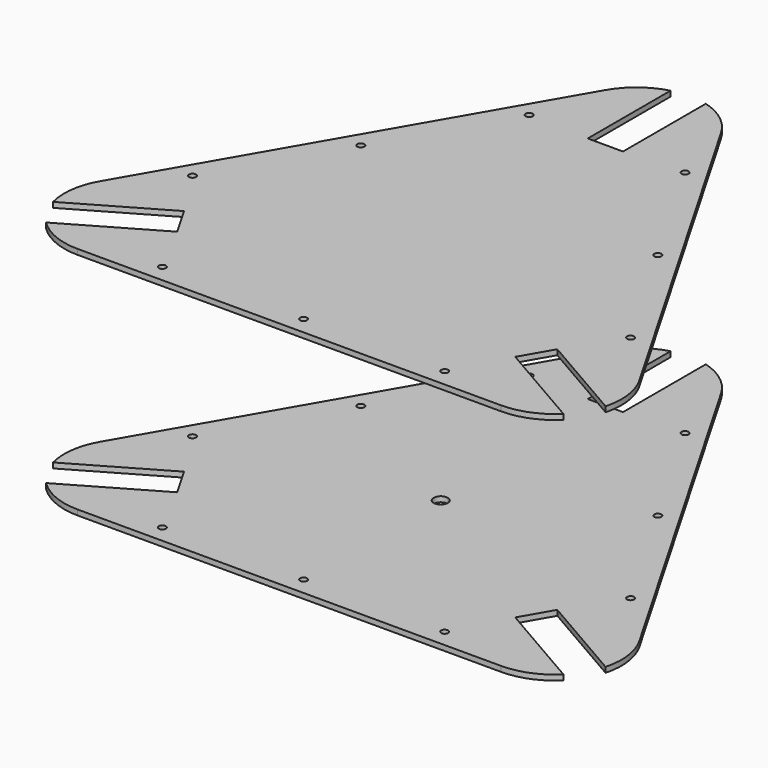
from build123d import *

# Parameters (mm, degrees)
F0_R     = 2
F0_R_2   = 4
F0_W     = 240
F0_H     = 20
F1_DEPTH = 3
F3_DEPTH = 3


# Not quite as in the source:
# - a feature names something its author has since deleted; it is built from what else it names


with BuildPart() as f1:
    # F0 (on Top) → F1 (new body)
    with BuildSketch(Plane.XY):
        Polygon((135.5000008485, -60.3331046), (152.8205089242, -50.3331046), (32.8205089242, 157.5129923082), (15.5000008485, 147.5129923082), align=None)
        with Locations((124.1602548864, -20.6920884487)):
            Circle(F0_R, mode=Mode.SUBTRACT)
        with Locations((84.1602548864, 48.5899438541)):
            Circle(F0_R, mode=Mode.SUBTRACT)
        with Locations((44.1602548864, 117.8719761568)):
            Circle(F0_R, mode=Mode.SUBTRACT)
        Polygon((-32.8205072271, 157.5129952477), (-152.8205072271, -50.3331016606), (-135.4999991515, -60.3331016606), (-15.4999991515, 147.5129952477), align=None)
        with Locations((-124.1602531893, -20.6920855092)):
            Circle(F0_R, mode=Mode.SUBTRACT)
        with Locations((-84.1602531893, 48.5899467935)):
            Circle(F0_R, mode=Mode.SUBTRACT)
        with Locations((-44.1602531893, 117.8719790963)):
            Circle(F0_R, mode=Mode.SUBTRACT)
        with BuildLine():
            Line((-120.0000016971, -107.1798906476), (-120.0000016971, -87.1798906476))
            Line((-120.0000016971, -87.1798906476), (119.9999983029, -87.1798906476))
            Line((119.9999983029, -87.1798906476), (119.9999983029, -107.1798906476))
            ThreePointArc((119.9999983029, -107.1798906476), (134.3544122401, -104.3562188159), (146.5698048192, -96.3059699854))
            Line((146.5698048192, -96.3059699854), (95.7997276302, -66.9938522536))
            Line((95.7997276302, -66.9938522536), (105.7997276302, -49.6733441779))
            Line((105.7997276302, -49.6733441779), (156.6259599909, -79.0178831132))
            ThreePointArc((156.6259599909, -79.0178831132), (157.5686990784, -64.2980017881), (152.8205089242, -50.3331046))
            Line((152.8205089242, -50.3331046), (135.5000008485, -60.3331046))
            Line((135.5000008485, -60.3331046), (15.5000008485, 147.5129923082))
            Line((15.5000008485, 147.5129923082), (32.8205089242, 157.5129923082))
            ThreePointArc((32.8205089242, 157.5129923082), (23.1979304174, 168.5324435184), (10.1185141338, 175.0861593938))
            Line((10.1185141338, 175.0861593938), (10.1185141338, 116.4619239302))
            Line((10.1185141338, 116.4619239302), (-9.8814858662, 116.4619239302))
            Line((-9.8814858662, 116.4619239302), (-9.8814858662, 175.1510018008))
            ThreePointArc((-9.8814858662, 175.1510018008), (-23.1006465781, 168.6074971372), (-32.8205072271, 157.5129952477))
            Line((-32.8205072271, 157.5129952477), (-15.4999991515, 147.5129952477))
            Line((-15.4999991515, 147.5129952477), (-135.4999991515, -60.3331016606))
            Line((-135.4999991515, -60.3331016606), (-152.8205072271, -50.3331016606))
            ThreePointArc((-152.8205072271, -50.3331016606), (-157.5523414703, -64.1762244295), (-156.6883173198, -78.7801884655))
            Line((-156.6883173198, -78.7801884655), (-105.9182417641, -49.4680716766))
            Line((-105.9182417641, -49.4680716766), (-95.9182417641, -66.7885797523))
            Line((-95.9182417641, -66.7885797523), (-146.7444724884, -96.1331177429))
            ThreePointArc((-146.7444724884, -96.1331177429), (-134.4680516673, -104.3094944517), (-120.0000016971, -107.1798906476))
        make_face()
        Circle(F0_R_2, mode=Mode.SUBTRACT)
        with Locations((-1.6971e-06, -97.1798906476)):
            Rectangle(F0_W, F0_H)
        with Locations((-80.0000016971, -97.1798906476)):
            Circle(F0_R, mode=Mode.SUBTRACT)
        with Locations((-1.6971e-06, -97.1798906476)):
            Circle(F0_R, mode=Mode.SUBTRACT)
        with Locations((79.9999983029, -97.1798906476)):
            Circle(F0_R, mode=Mode.SUBTRACT)
    extrude(amount=F1_DEPTH)


with BuildPart() as f1_1:
    # F2: moved
    add(f1.part.moved(Location((0, 0, -130))))


with BuildPart() as f3:
    # F0 (on Top) → F3 (new body)
    with BuildSketch(Plane.XY):
        with BuildLine():
            Line((-120.0000016971, -107.1798906476), (-120.0000016971, -87.1798906476))
            Line((-120.0000016971, -87.1798906476), (119.9999983029, -87.1798906476))
            Line((119.9999983029, -87.1798906476), (119.9999983029, -107.1798906476))
            ThreePointArc((119.9999983029, -107.1798906476), (134.3544122401, -104.3562188159), (146.5698048192, -96.3059699854))
            Line((146.5698048192, -96.3059699854), (95.7997276302, -66.9938522536))
            Line((95.7997276302, -66.9938522536), (105.7997276302, -49.6733441779))
            Line((105.7997276302, -49.6733441779), (156.6259599909, -79.0178831132))
            ThreePointArc((156.6259599909, -79.0178831132), (157.5686990784, -64.2980017881), (152.8205089242, -50.3331046))
            Line((152.8205089242, -50.3331046), (135.5000008485, -60.3331046))
            Line((135.5000008485, -60.3331046), (15.5000008485, 147.5129923082))
            Line((15.5000008485, 147.5129923082), (32.8205089242, 157.5129923082))
            ThreePointArc((32.8205089242, 157.5129923082), (23.1979304174, 168.5324435184), (10.1185141338, 175.0861593938))
            Line((10.1185141338, 175.0861593938), (10.1185141338, 116.4619239302))
            Line((10.1185141338, 116.4619239302), (-9.8814858662, 116.4619239302))
            Line((-9.8814858662, 116.4619239302), (-9.8814858662, 175.1510018008))
            ThreePointArc((-9.8814858662, 175.1510018008), (-23.1006465781, 168.6074971372), (-32.8205072271, 157.5129952477))
            Line((-32.8205072271, 157.5129952477), (-15.4999991515, 147.5129952477))
            Line((-15.4999991515, 147.5129952477), (-135.4999991515, -60.3331016606))
            Line((-135.4999991515, -60.3331016606), (-152.8205072271, -50.3331016606))
            ThreePointArc((-152.8205072271, -50.3331016606), (-157.5523414703, -64.1762244295), (-156.6883173198, -78.7801884655))
            Line((-156.6883173198, -78.7801884655), (-105.9182417641, -49.4680716766))
            Line((-105.9182417641, -49.4680716766), (-95.9182417641, -66.7885797523))
            Line((-95.9182417641, -66.7885797523), (-146.7444724884, -96.1331177429))
            ThreePointArc((-146.7444724884, -96.1331177429), (-134.4680516673, -104.3094944517), (-120.0000016971, -107.1798906476))
        make_face()
        Circle(F0_R_2, mode=Mode.SUBTRACT)
        with Locations((-1.6971e-06, -97.1798906476)):
            Rectangle(F0_W, F0_H)
        with Locations((-80.0000016971, -97.1798906476)):
            Circle(F0_R, mode=Mode.SUBTRACT)
        with Locations((-1.6971e-06, -97.1798906476)):
            Circle(F0_R, mode=Mode.SUBTRACT)
        with Locations((79.9999983029, -97.1798906476)):
            Circle(F0_R, mode=Mode.SUBTRACT)
        Polygon((-32.8205072271, 157.5129952477), (-152.8205072271, -50.3331016606), (-135.4999991515, -60.3331016606), (-15.4999991515, 147.5129952477), align=None)
        with Locations((-124.1602531893, -20.6920855092)):
            Circle(F0_R, mode=Mode.SUBTRACT)
        with Locations((-84.1602531893, 48.5899467935)):
            Circle(F0_R, mode=Mode.SUBTRACT)
        with Locations((-44.1602531893, 117.8719790963)):
            Circle(F0_R, mode=Mode.SUBTRACT)
        Polygon((135.5000008485, -60.3331046), (152.8205089242, -50.3331046), (32.8205089242, 157.5129923082), (15.5000008485, 147.5129923082), align=None)
        with Locations((124.1602548864, -20.6920884487)):
            Circle(F0_R, mode=Mode.SUBTRACT)
        with Locations((84.1602548864, 48.5899438541)):
            Circle(F0_R, mode=Mode.SUBTRACT)
        with Locations((44.1602548864, 117.8719761568)):
            Circle(F0_R, mode=Mode.SUBTRACT)
        Circle(F0_R_2)
    extrude(amount=F3_DEPTH)


solid = Compound([f1_1.part, f3.part])
